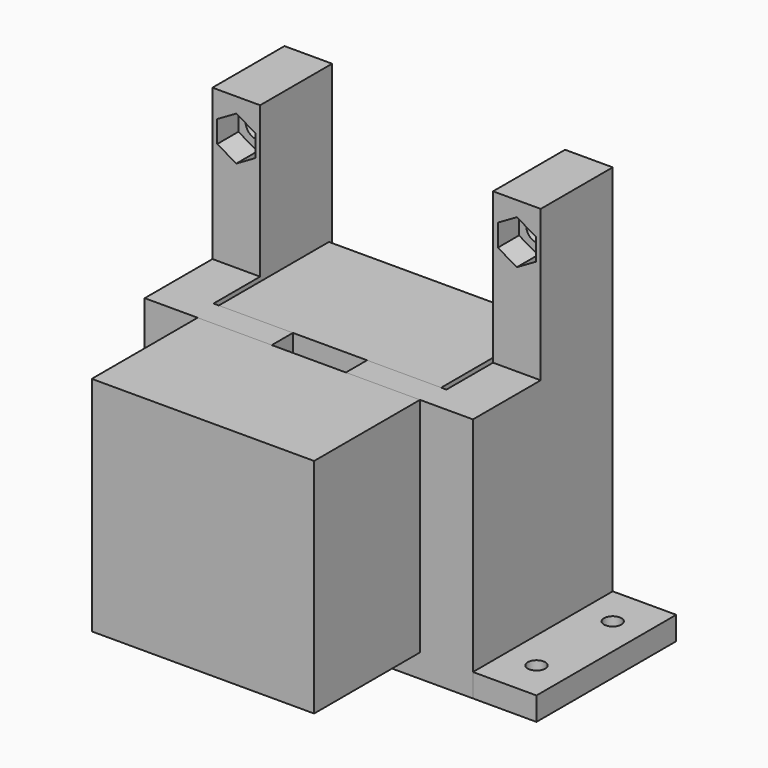
from build123d import *

# Parameters (mm, degrees)
F1_R      = 2.25
F2_DEPTH  = 12
F4_DEPTH  = 5
F5_W      = 44
F5_H      = 11
F5_H_2    = 5
F6_DEPTH  = 7
F7_DEPTH  = 42
F8_R      = 1.7
F8_R_2    = 13
F9_DEPTH  = 5
F11_REACH = 63.8670687473
F12_R     = 1.7
F13_DEPTH = 26
F14_W     = 42
F14_H     = 42
F14_R     = 1.7
F14_R_2   = 13
F15_DEPTH = 25
F19_DEPTH = 2.6
F20_W     = 12
F20_H     = 33
F21_DEPTH = 4.4
F22_D     = 3.3


with BuildPart() as f2:
    # F1 (on Front) → F2 (new body)
    with BuildSketch(Plane.XZ):
        Polygon((-27, 56.5), (-36, 56.5), (-36, -21), (26, -21), (26, 56.5), (17, 56.5), (17, -14), (-27, -14), align=None)
        with Locations((-31.5, 49.5)):
            Circle(F1_R, mode=Mode.SUBTRACT)
        with Locations((21.5, 49.5)):
            Circle(F1_R, mode=Mode.SUBTRACT)
    extrude(amount=-F2_DEPTH)

    # F3 (on face) → F4 (join)
    with BuildSketch(Plane.XZ):
        Polygon((-27, -14), (-27, 56.5), (-36, 56.5), (-36, -21), (26, -21), (26, 56.5), (17, 56.5), (17, -14), align=None)
        Polygon((-31.5, 53.6569219382), (-27.9, 51.5784609691), (-27.9, 47.4215390309), (-31.5, 45.3430780618), (-35.1, 47.4215390309), (-35.1, 51.5784609691), align=None, mode=Mode.SUBTRACT)
        Polygon((21.5, 53.6569219382), (25.1, 51.5784609691), (25.1, 47.4215390309), (21.5, 45.3430780618), (17.9, 47.4215390309), (17.9, 51.5784609691), align=None, mode=Mode.SUBTRACT)
    extrude(amount=F4_DEPTH)

    # F5 (on face) → F6 (join, through all)
    with BuildSketch(Plane.XY.offset(-14)):
        with Locations((-5, -10.5)):
            Rectangle(F5_W, F5_H)
        with Locations((-5, -18.5)):
            Rectangle(F5_W, F5_H_2)
        Polygon((-27, -16), (-27, -5), (-36, -5), (-36, -21), (-27, -21), align=None)
        Polygon((26, -5), (17, -5), (17, -16), (17, -21), (26, -21), align=None)
    extrude(amount=-F6_DEPTH)

    # F5 (on face) → F7 (join)
    with BuildSketch(Plane.XY.offset(-14)):
        with Locations((-5, -18.5)):
            Rectangle(F5_W, F5_H_2)
        Polygon((-27, -16), (-27, -5), (-36, -5), (-36, -21), (-27, -21), align=None)
        Polygon((26, -5), (17, -5), (17, -16), (17, -21), (26, -21), align=None)
    extrude(amount=F7_DEPTH)

    # F8 (on face) → F9 (cut, through all)
    with BuildSketch(Plane.XZ.offset(21)):
        with Locations((-20.5, 22.5)):
            Circle(F8_R)
        with Locations((-5, 7)):
            Circle(F8_R_2)
        with Locations((-20.5, -8.5)):
            Circle(F8_R)
        with Locations((10.5, -8.5)):
            Circle(F8_R)
        with Locations((10.5, 22.5)):
            Circle(F8_R)
    extrude(amount=-F9_DEPTH, mode=Mode.SUBTRACT)

    f11_end = f2.faces().sort_by_distance((-18, -18.5, 7))[0]
    # F10 (on face) → F11 (cut, up to a face of the model that its end follows)
    with BuildSketch(Plane.XY.offset(28)):
        Polygon((2, -16), (-5, -16), (-12, -16), (-12, -21), (2, -21), align=None)
    f11_long = extrude(amount=-F11_REACH, mode=Mode.PRIVATE)
    add(split(f11_long, bisect_by=f11_end, keep=Keep.ALL, mode=Mode.PRIVATE).solids().sort_by_distance((-5, -18.5, 28))[0], mode=Mode.SUBTRACT)

    # F19 (cut, through all): a face of the model
    f19_faces = [f2.faces().sort_by_distance(p)[0] for p in [
        (-5, -4.5, -21),
    ]]
    extrude(f19_faces, amount=-F19_DEPTH, mode=Mode.SUBTRACT)


with BuildPart() as f13:
    # F12 (on face) → F13 (new body)
    with BuildSketch(Plane(origin=(0, -16, 0), x_dir=(-1, 0, 0), z_dir=(0, 1, 0))):
        with BuildLine():
            Line((-16, -14), (26, -14))
            Line((26, -14), (26, 28))
            Line((26, 28), (12, 28))
            Line((12, 28), (12, 17.9544511501))
            ThreePointArc((12, 17.9544511501), (5, -6), (-2, 17.9544511501))
            Line((-2, 17.9544511501), (-2, 28))
            Line((-2, 28), (-16, 28))
            Line((-16, 28), (-16, -14))
        make_face()
        with Locations((-10.5, -8.5)):
            Circle(F12_R, mode=Mode.SUBTRACT)
        with Locations((20.5, -8.5)):
            Circle(F12_R, mode=Mode.SUBTRACT)
        with Locations((-10.5, 22.5)):
            Circle(F12_R, mode=Mode.SUBTRACT)
        with Locations((20.5, 22.5)):
            Circle(F12_R, mode=Mode.SUBTRACT)
        with BuildLine():
            Line((12, 17.9544511501), (12, 28))
            Line((12, 28), (-2, 28))
            Line((-2, 28), (-2, 17.9544511501))
            ThreePointArc((-2, 17.9544511501), (5, -6), (12, 17.9544511501))
        make_face()
        with Locations((-10.5, 22.5)):
            Circle(F12_R)
        with Locations((20.5, 22.5)):
            Circle(F12_R)
        with Locations((-10.5, -8.5)):
            Circle(F12_R)
        with Locations((20.5, -8.5)):
            Circle(F12_R)
    extrude(amount=F13_DEPTH)


with BuildPart() as f15:
    # F14 (on face) → F15 (new body)
    with BuildSketch(Plane.XZ.offset(21)):
        with Locations((-5, 7)):
            Rectangle(F14_W, F14_H)
        with Locations((-20.5, -8.5)):
            Circle(F14_R, mode=Mode.SUBTRACT)
        with Locations((10.5, -8.5)):
            Circle(F14_R, mode=Mode.SUBTRACT)
        with Locations((-20.5, 22.5)):
            Circle(F14_R, mode=Mode.SUBTRACT)
        with Locations((-5, 7)):
            Circle(F14_R_2, mode=Mode.SUBTRACT)
        with Locations((10.5, 22.5)):
            Circle(F14_R, mode=Mode.SUBTRACT)
    extrude(amount=F15_DEPTH)

    # F8 (on face) → F15, piece 2 (join)
    with BuildSketch(Plane.XZ.offset(21)):
        with Locations((-20.5, 22.5)):
            Circle(F8_R)
    extrude(amount=F15_DEPTH)

    # F8 (on face) → F15, piece 3 (join)
    with BuildSketch(Plane.XZ.offset(21)):
        with Locations((-5, 7)):
            Circle(F8_R_2)
    extrude(amount=F15_DEPTH)

    # F8 (on face) → F15, piece 4 (join)
    with BuildSketch(Plane.XZ.offset(21)):
        with Locations((-20.5, -8.5)):
            Circle(F8_R)
    extrude(amount=F15_DEPTH)

    # F8 (on face) → F15, piece 5 (join)
    with BuildSketch(Plane.XZ.offset(21)):
        with Locations((10.5, 22.5)):
            Circle(F8_R)
    extrude(amount=F15_DEPTH)

    # F8 (on face) → F15, piece 6 (join)
    with BuildSketch(Plane.XZ.offset(21)):
        with Locations((10.5, -8.5)):
            Circle(F8_R)
    extrude(amount=F15_DEPTH)


with BuildPart() as f21:
    # F20 (on face) → F21 (new body, through all)
    with BuildSketch(Plane(origin=(0, 0, -18.4), x_dir=(1, 0, 0), z_dir=(0, 0, -1))):
        with Locations((32, 4.5)):
            Rectangle(F20_W, F20_H)
    extrude(amount=-F21_DEPTH)

    # F22 (through all)
    with Locations(Plane(origin=(0, 0, -18.4), x_dir=(1, 0, 0), z_dir=(0, 0, -1))):
        with Locations((32, -4.5), (32, 13.5)):
            Hole(F22_D / 2)


solid = Compound([f2.part, f13.part, f15.part, f21.part])
